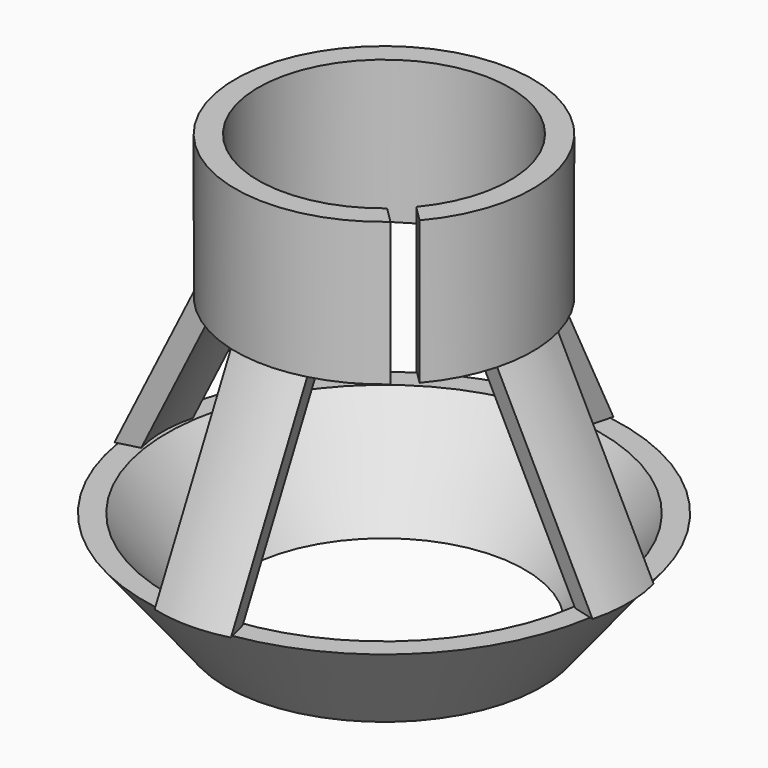
from build123d import *

# Parameters (mm, degrees)
F1_DEPTH        = 19.05
F4_COPIES_COUNT = 4


# Not quite as in the source:
# - a pattern or mirror of a feature is missing from the dataset's text; its kind, count and spacing are read off the source's solid


with BuildPart() as f1:
    # F0 (on Top) → F1 (new body)
    with BuildSketch(Plane.XY):
        with BuildLine():
            ThreePointArc((10.71820488, -12.8734663491), (-11.8449578237, 11.8449578237), (12.8734663491, -10.71820488))
            Line((12.8734663491, -10.71820488), (15.0363144921, -12.8810530231))
            ThreePointArc((15.0363144921, -12.8810530231), (-14.0002192927, 14.0002192927), (12.8810530231, -15.0363144921))
            Line((12.8810530231, -15.0363144921), (10.71820488, -12.8734663491))
        make_face()
    extrude(amount=F1_DEPTH)

    # F4: sweep along a path in F3
    with BuildLine(Plane.YZ) as f4_path:
        Line((-32.4993, -25.4), (-19.7993, 0))
    # F2 (on face) → F4 (sweep)
    with BuildSketch(Plane(origin=(0, 0, 0), x_dir=(1, 0, 0), z_dir=(0, 0, -1))):
        with BuildLine():
            ThreePointArc((5.08, 19.136506486), (0, 19.7993), (-5.08, 19.136506486))
            Line((-5.08, 19.136506486), (-4.2979602309, 16.1905401251))
            ThreePointArc((-4.2979602309, 16.1905401251), (0, 16.7513), (4.2979602309, 16.1905401251))
            Line((4.2979602309, 16.1905401251), (5.08, 19.136506486))
        make_face()
    f4 = sweep(path=f4_path.line)

    # F4_copies: F4 ×4 about axis
    f4_copies_axis = Axis((0, 0, 0), (0, 0, 1))
    for i in range(1, F4_COPIES_COUNT):
        add(f4.rotate(f4_copies_axis, i * 360 / F4_COPIES_COUNT))

    # F7 (on Right) → F8 (revolve)
    with BuildSketch(Plane.YZ):
        Polygon((-18.7305401251, -38.1), (-28.8905401251, -25.4), (-31.836506486, -25.4), (-20.986948621, -38.9619473312), align=None)
    revolve(axis=Axis((0, 0, -16.1163), (0, 0, -1)))


solid = f1.part
